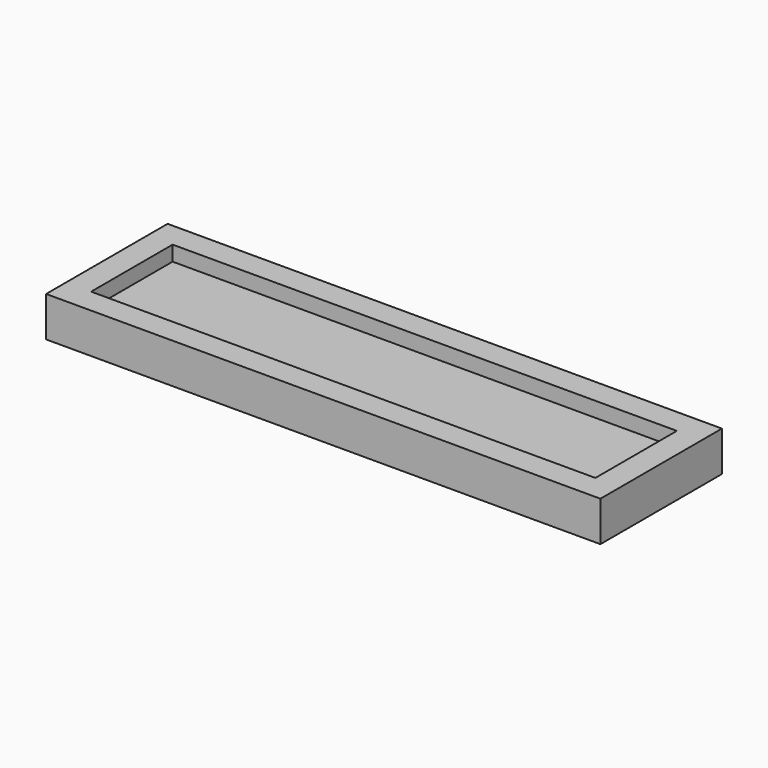
from build123d import *

# Parameters (mm, degrees)
F0_W     = 56.261
F0_H     = 15.4178
F0_W_2   = 51.181
F0_H_2   = 10.3378
F1_DEPTH = 1.27
F2_DEPTH = 2.794


# Not quite as in the source:
# - a feature names something its author has since deleted; it is built from what else it names


with BuildPart() as f1:
    # F0 (on Top) → F1 (new body, symmetric)
    with BuildSketch(Plane.XY):
        Rectangle(F0_W, F0_H)
        Rectangle(F0_W_2, F0_H_2, mode=Mode.SUBTRACT)
        Rectangle(F0_W_2, F0_H_2)
    extrude(amount=F1_DEPTH, both=True)

    # F0 (on Top) → F2 (join)
    with BuildSketch(Plane.XY):
        Rectangle(F0_W, F0_H)
        Rectangle(F0_W_2, F0_H_2, mode=Mode.SUBTRACT)
    extrude(amount=F2_DEPTH)


solid = f1.part
